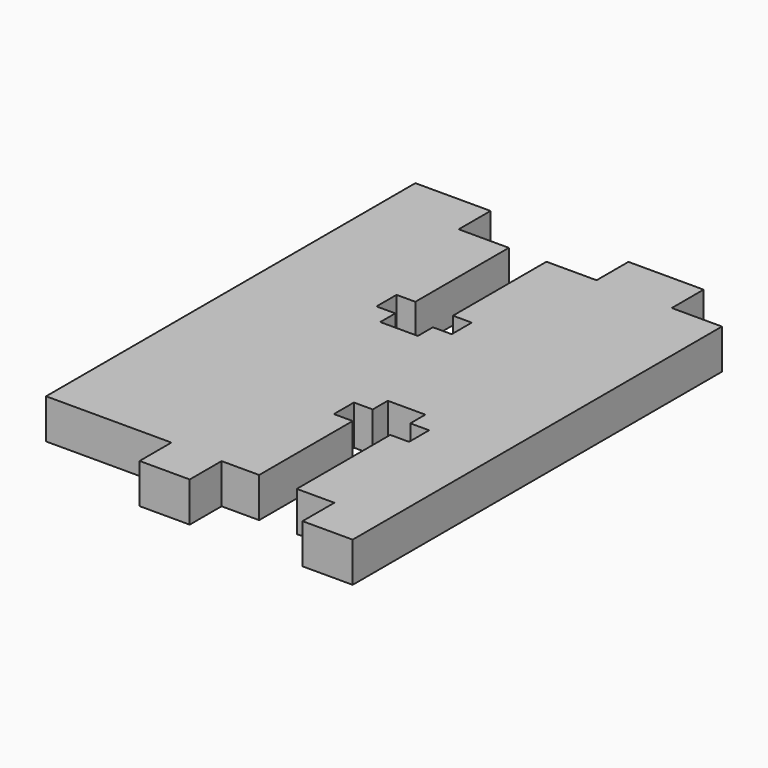
from build123d import *

# Parameters (mm, degrees)
F0_W     = 6
F0_H     = 3.175
F0_W_2   = 4
F1_DEPTH = 3.175


# Not quite as in the source:
# - a length typed as a fraction of an inch, garbled in the dataset ("3 / 203.2 mm" for 3/8 in), is restored


with BuildPart() as f1:
    # F0 (on Top) → F1 (new body)
    with BuildSketch(Plane.XY):
        Polygon((-26.613304615, 17.7200174183), (-26.613304615, 27.0450174183), (-30.613304615, 27.0450174183), (-36.613304615, 27.0450174183), (-36.613304615, -6.6049825817), (-26.613304615, -6.6049825817), (-22.613304615, -6.6049825817), (-19.613304615, -6.6049825817), (-19.613304615, 2.7200174183), (-21.113304615, 2.7200174183), (-21.113304615, 4.7200174183), (-19.613304615, 4.7200174183), (-19.613304615, 6.2200174183), (-16.613304615, 6.2200174183), (-16.613304615, 4.7200174183), (-15.113304615, 4.7200174183), (-15.113304615, 2.7200174183), (-16.613304615, 2.7200174183), (-16.613304615, -6.6049825817), (-13.613304615, -6.6049825817), (-9.613304615, -6.6049825817), (-9.613304615, 27.0450174183), (-13.613304615, 27.0450174183), (-19.613304615, 27.0450174183), (-23.613304615, 27.0450174183), (-23.613304615, 17.7200174183), (-22.113304615, 17.7200174183), (-22.113304615, 15.7200174183), (-23.613304615, 15.7200174183), (-23.613304615, 14.2200174183), (-26.613304615, 14.2200174183), (-26.613304615, 15.7200174183), (-28.113304615, 15.7200174183), (-28.113304615, 17.7200174183), align=None)
        with Locations((-33.613304615, 28.6325174183)):
            Rectangle(F0_W, F0_H)
        with Locations((-16.613304615, 28.6325174183)):
            Rectangle(F0_W, F0_H)
        with Locations((-24.613304615, -8.1924825817)):
            Rectangle(F0_W_2, F0_H)
        with Locations((-11.613304615, -8.1924825817)):
            Rectangle(F0_W_2, F0_H)
    extrude(amount=F1_DEPTH)


solid = f1.part
